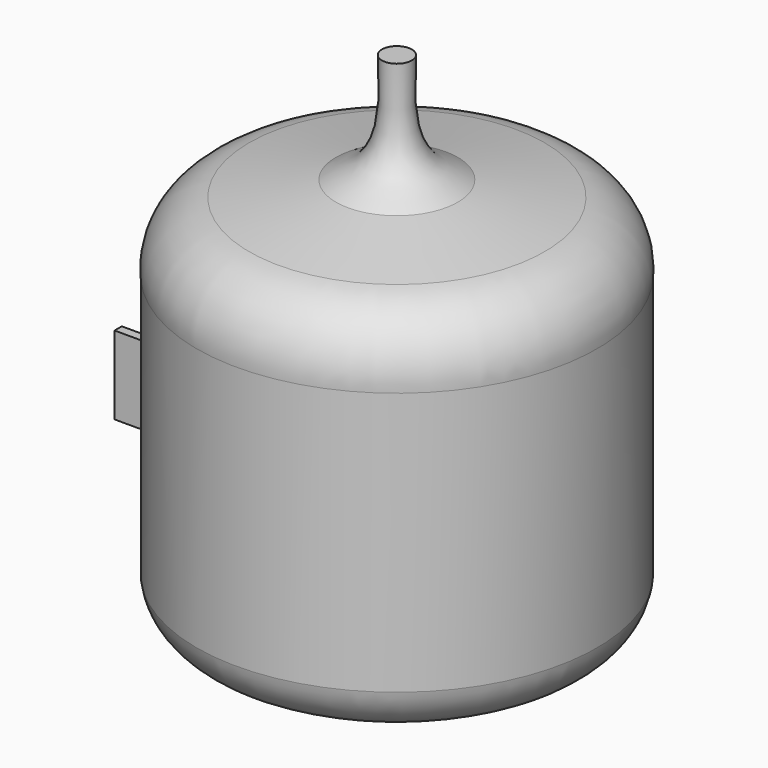
from build123d import *

# Parameters (mm, degrees)
F4_TEXT_SIZE = 20.9098371367
F5_DEPTH     = 25.4


# Not quite as in the source:
# - Text() gives the source's letters only with a copy of the font that has no kerning and outlines rounded to 1/6400 em; it was checked with that copy


with BuildPart() as f2:
    # F0 (on Front) → F2 (revolve)
    with BuildSketch(Plane.XZ):
        with BuildLine():
            Line((-26.5051375575, 0), (0, 0))
            Line((0, 0), (0, 96.0873439908))
            Line((0, 96.0873439908), (-2.8516349848, 96.0873439908))
            add(Edge.make_bspline(
                [(-11.6173978895, 75.1393735409), (-9.7426347568, 76.3456312385), (-5.3043791323, 77.8458976859), (-2.4444916933, 85.4503779773), (-2.6816550821, 92.2637685262), (-2.8516349848, 96.0873439908)],
                knots=[0, 0, 0, 0, 0.2985909834, 0.6144739767, 1, 1, 1, 1], degree=3))
            Line((-11.6173978895, 75.1393735409), (-28.1655207627, 72.2003063953))
            ThreePointArc((-28.1655207627, 72.2003063953), (-35.7011013622, 67.619179053), (-38.1691418588, 59.1527465809))
            Line((-38.1691418588, 59.1527465809), (-38.1691418588, 8.9668690974))
            ThreePointArc((-38.1691418588, 8.9668690974), (-34.1775154482, 2.0894941092), (-26.5051375575, 0))
        make_face()
    revolve(axis=Axis((0, 0, 44.9557676911), (0, 0, -1)))

    # F4 (on offset) → F5 (join)
    with BuildSketch(Plane.YZ.offset(-40.64)):
        with Locations((-18.547931686, 28.387799859)):
            Text('H2O', F4_TEXT_SIZE, font='Open Sans', text_align=(TextAlign.LEFT, TextAlign.BOTTOM))
    extrude(amount=F5_DEPTH)


solid = f2.part
